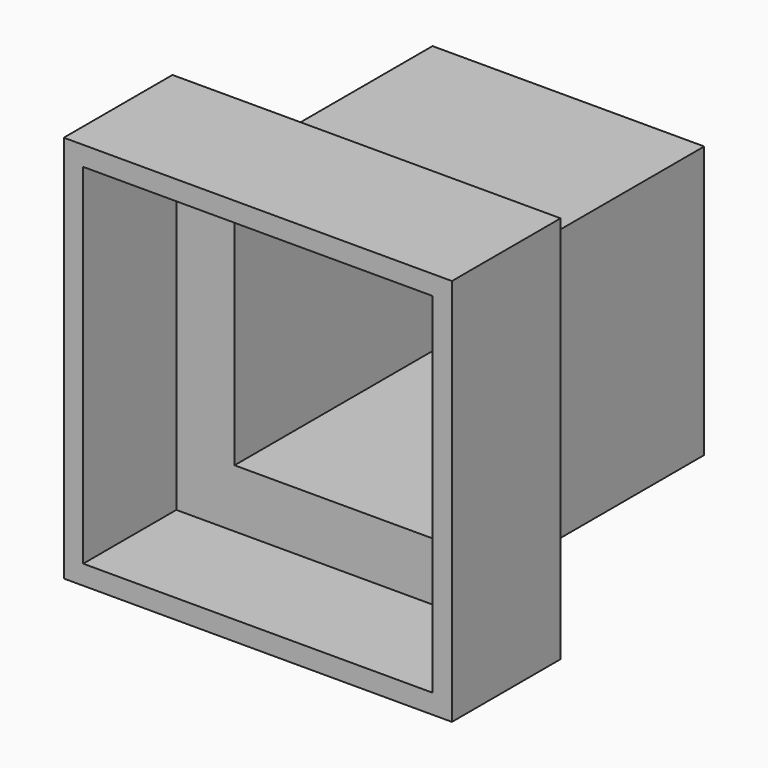
from build123d import *

# Parameters (mm, degrees)
F10_W     = 100
F10_H     = 100
F14_DEPTH = 35
F13_W     = 70
F13_H     = 70
F15_DEPTH = 65
F16_T     = -5
F21_D     = 25.4


# Not quite as in the source:
# - the program builds the solid bodies; features that only make, move or delete a surface that nothing else refers to are left out


with BuildPart() as f14:
    # F10 (on offset) → F14 (new body, through all)
    with BuildSketch(Plane.XZ.offset(-406.68448)):
        with Locations((37.5531539321, 417.7168309689)):
            Rectangle(F10_W, F10_H)
    extrude(amount=-F14_DEPTH)

    # F13 (on offset) → F15 (join, through all)
    with BuildSketch(Plane.XZ.offset(-506.68448)):
        with Locations((37.5531539321, 417.7168309689)):
            Rectangle(F13_W, F13_H)
    extrude(amount=F15_DEPTH)

    # F16
    f16_openings = [f14.faces().sort_by_distance(p)[0] for p in [
        (37.553154, 406.68448, 417.716831),
    ]]
    offset(amount=F16_T, openings=f16_openings, kind=Kind.INTERSECTION)

    # F21 (through all)
    with Locations(Plane.XZ.offset(-441.68448)):
        with Locations((37.5531539321, 417.7168309689)):
            Hole(F21_D / 2)


solid = f14.part
